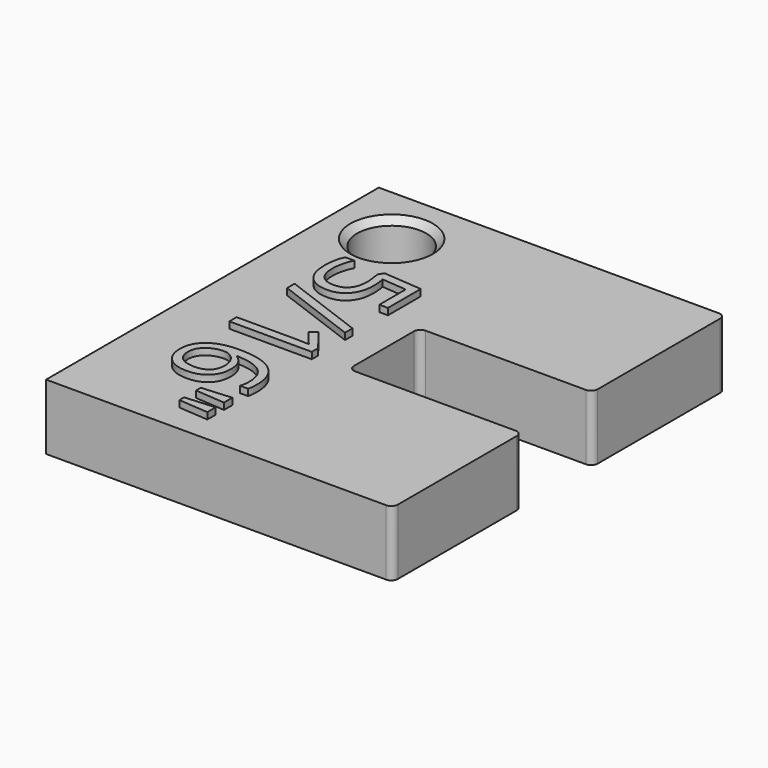
from build123d import *

# Parameters (mm, degrees)
F0_R         = 3.175
F1_DEPTH     = 6
F2_R         = 0.6
F3_SIZE      = 0.6
F4_TEXT_SIZE = 10.5833333333
F5_DEPTH     = 0.6


# Not quite as in the source:
# - Text() gives the source's letters only with a copy of the font that has no kerning and outlines rounded to 1/6400 em; it was checked with that copy


with BuildPart() as f1:
    # F0 (on Top) → F1 (new body)
    with BuildSketch(Plane.XY):
        Polygon((10.0186250234, 28.5263651589), (-21.7313749766, 28.5263651589), (-21.7313749766, -9.5736348411), (10.0186250234, -9.5736348411), (10.0186250234, 5.230821153), (-5.8563749766, 5.230821153), (-5.8563749766, 13.308021153), (10.0186250234, 13.308021153), align=None)
        with Locations((-16.0552702235, 22.9080564802)):
            Circle(F0_R, mode=Mode.SUBTRACT)
    extrude(amount=F1_DEPTH)

    # F2
    f2_edges = [f1.edges().sort_by_distance(p)[0] for p in [
        (10.018625, -9.573635, 3),
        (10.018625, 5.230821, 3),
        (10.018625, 13.308021, 3),
        (-5.856375, 13.308021, 3),
        (-5.856375, 5.230821, 3),
        (10.018625, 28.526365, 3),
    ]]
    fillet(f2_edges, radius=F2_R)

    # F3
    f3_edges = [f1.edges().sort_by_distance(p)[0] for p in [
        (-19.23027, 22.908056, 6),
        (-19.23027, 22.908056, 0),
    ]]
    chamfer(f3_edges, length=F3_SIZE)

    # F4 (on face) → F5 (join)
    with BuildSketch(Plane.XY.offset(6)):
        with Locations(Location((-16.4102533934, 18.3892877524), (0, 0, -90))):
            Text('5/16"', F4_TEXT_SIZE, font='Open Sans', text_align=(TextAlign.LEFT, TextAlign.BOTTOM))
    extrude(amount=F5_DEPTH)


solid = f1.part
